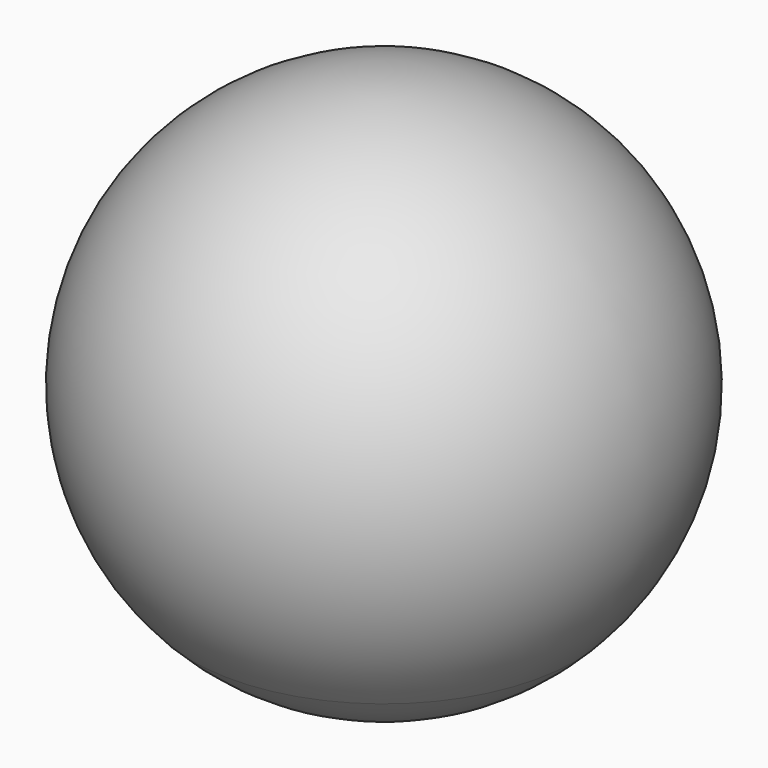
from build123d import *

# Parameters (mm, degrees)
F5_DEPTH      = 2.138281953
F5_DEPTH_BACK = 11.6513629711


with BuildPart() as f1:
    # F0 (on Front) → F1 (revolve)
    with BuildSketch(Plane.XZ):
        with BuildLine():
            Line((1.75, 0), (4.99, 0))
            ThreePointArc((4.99, 0), (6.3370154126, 7.4707660014), (0, 11.6503629711))
            Line((0, 11.6503629711), (0, 11.3503629711))
            Line((0, 11.3503629711), (1.75, 10.34))
            Line((1.75, 10.34), (1.75, 0))
        make_face()
    revolve(axis=Axis((0, 0, 4.4251814855), (0, 0, 1)))


with BuildPart() as f2:
    # F0 (on Front) → F2 (revolve)
    with BuildSketch(Plane.XZ):
        with BuildLine():
            ThreePointArc((0, -2.137281953), (2.7142252185, -1.5804751024), (4.99, 0))
            Line((4.99, 0), (1.75, 0))
            Line((1.75, 0), (1.75, -0.8269189819))
            Line((1.75, -0.8269189819), (0, -1.837281953))
            Line((0, -1.837281953), (0, -2.137281953))
        make_face()
    revolve(axis=Axis((0, 0, 4.4251814855), (0, 0, 1)))


with BuildPart() as f3:
    # F0 (on Front) → F3 (revolve)
    with BuildSketch(Plane.XZ):
        Polygon((1.45, -0.6537139012), (1.45, 0), (1.45, 10.1667949192), (0, 11.0039528096), (0, -1.4908717915), align=None)
    revolve(axis=Axis((0, 0, 4.756540509), (0, 0, -1)))

    # F4 (on Top) → F5 (cut, two sides)
    with BuildSketch(Plane.XY) as f5_sk:
        with BuildLine():
            Line((0.9, -1.1368817001), (-0.9, -1.1368817001))
            ThreePointArc((-0.9, -1.1368817001), (0, -1.45), (0.9, -1.1368817001))
        make_face()
    extrude(amount=-F5_DEPTH, mode=Mode.SUBTRACT)
    extrude(f5_sk.sketch, amount=F5_DEPTH_BACK, mode=Mode.SUBTRACT)


solid = Compound([f1.part, f2.part, f3.part])
